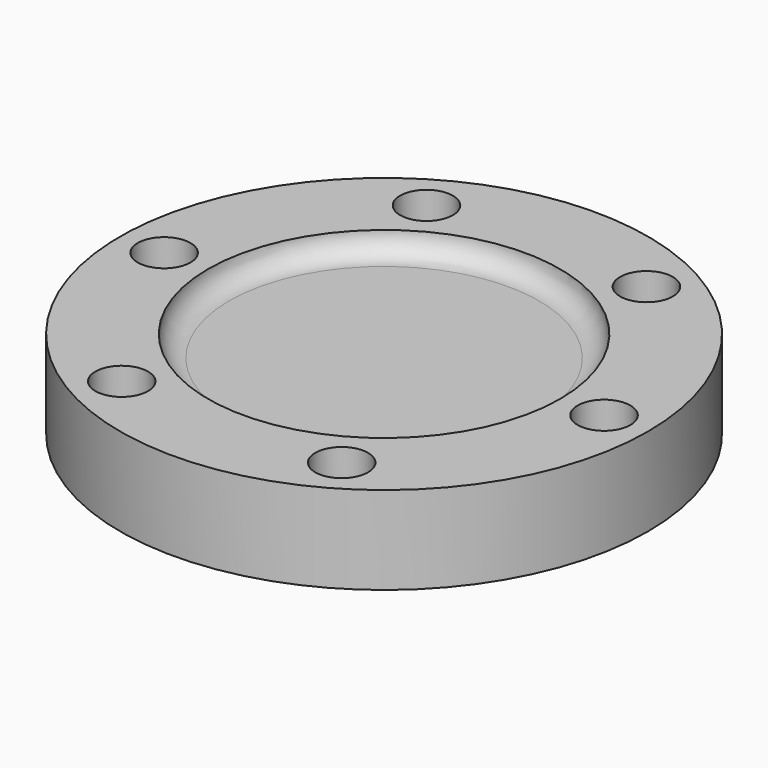
from build123d import *

# Parameters (mm, degrees)
F0_R     = 19.05
F1_DEPTH = 6.35
F2_D     = 3.81
F3_R     = 12.7
F4_DEPTH = 1.524
F5_R     = 1.52399


# Not quite as in the source:
# - a fillet or chamfer is up to 0.001 mm smaller than in the source, because OpenCascade refuses the exact size


with BuildPart() as f1:
    # F0 (on Top) → F1 (new body)
    with BuildSketch(Plane.XY):
        Circle(F0_R)
    extrude(amount=F1_DEPTH)

    # F2 (through all)
    with Locations(Plane(origin=(0, 0, 0), x_dir=(1, 0, 0), z_dir=(0, 0, -1))):
        with Locations((7.9375, 13.7481532851), (-7.9375, 13.7481532851), (-15.875, 0), (-7.9375, -13.7481532851), (7.9375, -13.7481532851), (15.875, 0)):
            Hole(F2_D / 2)

    # F3 (on face) → F4 (cut)
    with BuildSketch(Plane.XY.offset(6.35)):
        Circle(F3_R)
    extrude(amount=-F4_DEPTH, mode=Mode.SUBTRACT)

    # F5 (radius 1.524 in the source; OpenCascade refuses exactly that, so slightly less here)
    f5_edges = [f1.edges().sort_by_distance(p)[0] for p in [
        (-12.7, 0, 4.826),
    ]]
    fillet(f5_edges, radius=F5_R)


solid = f1.part
